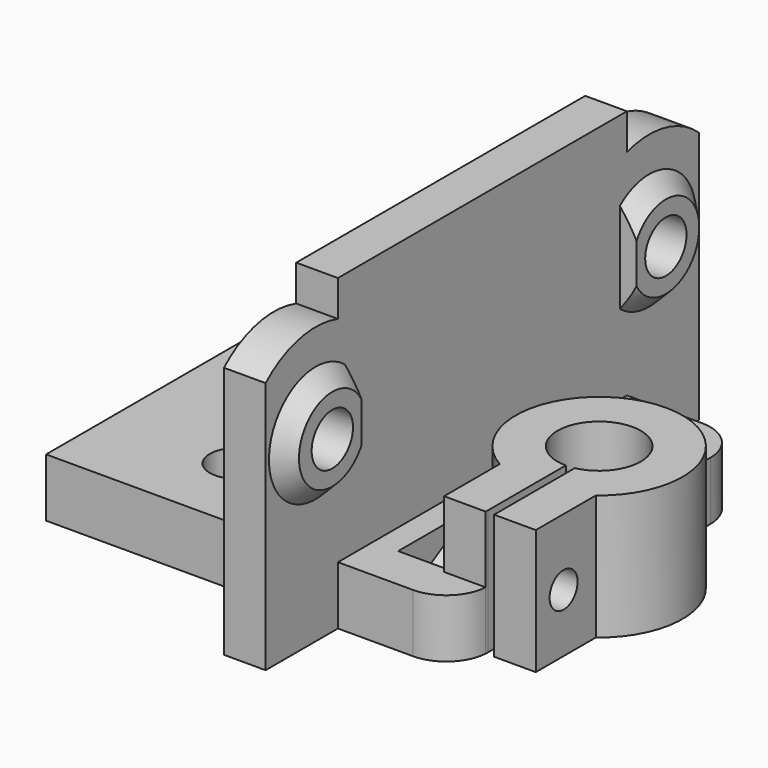
from build123d import *

# Parameters (mm, degrees)
F0_R          = 3.1
F1_DEPTH      = 7
F2_DEPTH      = 15
F4_DEPTH      = 2
F4_DEPTH_BACK = 6
F5_R          = 2.1
F6_DEPTH      = 25
F8_DEPTH      = 30
F9_DEPTH      = 25
F9_DEPTH_BACK = 7
F10_R         = 3.1
F11_DEPTH     = 25
F12_R         = 5
F12_R_2       = 3.1
F13_DEPTH     = 7
F14_SIZE      = 1.99999
F15_W         = 3.459926136
F15_H         = 15.633740799
F16_DEPTH     = 25
F18_DEPTH     = 25


# Not quite as in the source:
# - a fillet or chamfer is up to 0.001 mm smaller than in the source, because OpenCascade refuses the exact size


with BuildPart() as f1:
    # F0 (on Top) → F1 (new body)
    with BuildSketch(Plane.XY):
        with BuildLine():
            ThreePointArc((-5, -21.6602540378), (-1.5866973333, -20.3139323085), (-0.0115560862, -17))
            Line((-0.0115560862, -17), (-5, -17))
            Line((-5, -17), (-5, -8.6602540378))
            ThreePointArc((-5, -8.6602540378), (-9.6592582629, 2.588190451), (0, 10))
            Line((0, 10), (0, 16.6602540378))
            ThreePointArc((0, 16.6602540378), (-1.4644660941, 20.1957879438), (-5, 21.6602540378))
            Line((-5, 21.6602540378), (-49, 21.6602540378))
            Line((-49, 21.6602540378), (-49, 0))
            Line((-49, 0), (-49, -21.6602540378))
            Line((-49, -21.6602540378), (-5, -21.6602540378))
        make_face()
        with Locations((-34, -12)):
            Circle(F0_R, mode=Mode.SUBTRACT)
        with Locations((-34, 12)):
            Circle(F0_R, mode=Mode.SUBTRACT)
    extrude(amount=F1_DEPTH)

    # F0 (on Top) → F2 (join)
    with BuildSketch(Plane.XY):
        with BuildLine():
            ThreePointArc((0, -5), (-0.50254481, 4.974680765), (1, -4.8989794856))
            Line((1, -4.8989794856), (1, -9.9498743711))
            Line((1, -9.9498743711), (1, -17))
            Line((1, -17), (6, -17))
            Line((6, -17), (6, -8))
            ThreePointArc((6, -8), (9.4868329805, 3.1622776602), (0, 10))
            ThreePointArc((0, 10), (-9.6592582629, 2.588190451), (-5, -8.6602540378))
            Line((-5, -8.6602540378), (-5, -17))
            Line((-5, -17), (-0.0115560862, -17))
            ThreePointArc((-0.0115560862, -17), (-0.0028898567, -16.8302252574), (0, -16.6602540378))
            Line((0, -16.6602540378), (0, -10))
            Line((0, -10), (0, -5))
        make_face()
    extrude(amount=F2_DEPTH)

    # F3 (on face) → F4 (cut, two sides)
    with BuildSketch(Plane(origin=(-5, 0, 0), x_dir=(0, -1, 0), z_dir=(-1, 0, 0))) as f4_sk:
        Polygon((16.3801270189, 4.9504065444), (16.3801270189, 9.0495934556), (12.8301270189, 11.0991869112), (9.2801270189, 9.0495934556), (9.2801270189, 4.9504065444), (12.8301270189, 2.9008130888), align=None)
    extrude(amount=-F4_DEPTH, mode=Mode.SUBTRACT)
    extrude(f4_sk.sketch, amount=F4_DEPTH_BACK, mode=Mode.SUBTRACT)

    # F5 (on face) → F6 (cut)
    with BuildSketch(Plane(origin=(-5, 0, 0), x_dir=(0, -1, 0), z_dir=(-1, 0, 0))):
        with Locations((12.8301270189, 7)):
            Circle(F5_R)
    extrude(amount=-F6_DEPTH, mode=Mode.SUBTRACT)

    # F7 (on face) → F8 (join)
    with BuildSketch(Plane.XY.offset(7)):
        Polygon((-19, 32.5), (-19, 21.6602540378), (-19, -21.6602540378), (-19, -32.5), (-14, -32.5), (-14, -21.6602540378), (-14, 21.6602540378), (-14, 32.5), align=None)
    extrude(amount=F8_DEPTH)

    # F7 (on face) → F9 (join, two sides)
    with BuildSketch(Plane.XY.offset(7)) as f9_sk:
        Polygon((-19, 32.5), (-19, 21.6602540378), (-19, -21.6602540378), (-19, -32.5), (-14, -32.5), (-14, -21.6602540378), (-14, 21.6602540378), (-14, 32.5), align=None)
    extrude(amount=F9_DEPTH)
    extrude(f9_sk.sketch, amount=-F9_DEPTH_BACK)

    # F10 (on face) → F11 (cut)
    with BuildSketch(Plane(origin=(-19, 0, 0), x_dir=(0, -1, 0), z_dir=(-1, 0, 0))):
        with Locations((-25, 22)):
            Circle(F10_R)
        with Locations((25, 22)):
            Circle(F10_R)
    extrude(amount=-F11_DEPTH, mode=Mode.SUBTRACT)

    # F12 (on face) → F13 (join)
    with BuildSketch(Plane(origin=(-19, 0, 0), x_dir=(0, -1, 0), z_dir=(-1, 0, 0))):
        with Locations((25, 22)):
            Circle(F12_R)
        with Locations((25, 22)):
            Circle(F12_R_2, mode=Mode.SUBTRACT)
        with Locations((-25, 22)):
            Circle(F12_R)
        with Locations((-25, 22)):
            Circle(F12_R_2, mode=Mode.SUBTRACT)
    extrude(amount=-F13_DEPTH)

    # F14 (size 2 in the source; OpenCascade refuses exactly that, so slightly less here)
    f14_edges = [f1.edges().sort_by_distance(p)[0] for p in [
        (-14, 30, 22),
        (-14, -20, 22),
    ]]
    chamfer(f14_edges, length=F14_SIZE)

    # F15 (on face) → F16 (cut)
    with BuildSketch(Plane.YZ.offset(-14)):
        with Locations((18.870036932, 22.279205732)):
            Rectangle(F15_W, F15_H)
        with Locations((-18.870036932, 22.279205732)):
            Rectangle(F15_W, F15_H)
    extrude(amount=F16_DEPTH, mode=Mode.SUBTRACT)

    # F17 (on face) → F18 (cut)
    with BuildSketch(Plane.YZ.offset(-14)):
        with BuildLine():
            Line((21.6602540378, 43.2897545397), (21.6602540378, 32.6861559824))
            ThreePointArc((21.6602540378, 32.6861559824), (27.3948854866, 32.9367434036), (32.5, 30.3125106178))
            Line((32.5, 30.3125106178), (32.5, 43.2897545397))
            Line((32.5, 43.2897545397), (21.6602540378, 43.2897545397))
        make_face()
        with BuildLine():
            ThreePointArc((-32.5, 30.3125106178), (-27.3948854866, 32.9367434036), (-21.6602540378, 32.6861559824))
            Line((-21.6602540378, 32.6861559824), (-21.6602540378, 43.2897545397))
            Line((-21.6602540378, 43.2897545397), (-32.5, 43.2897545397))
            Line((-32.5, 43.2897545397), (-32.5, 30.3125106178))
        make_face()
    extrude(amount=-F18_DEPTH, mode=Mode.SUBTRACT)


solid = f1.part
